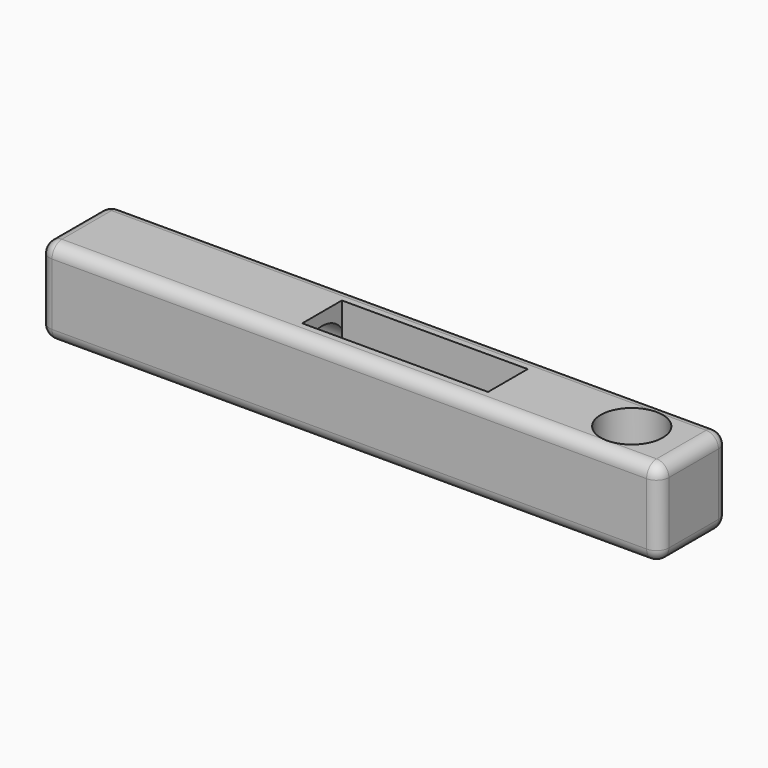
from build123d import *

# Parameters (mm, degrees)
F0_W     = 177.8
F0_H     = 177.8
F1_DEPTH = 1270
F2_R     = 63.5
F3_DEPTH = 177.8
F4_R     = 63.5
F5_DEPTH = 508
F6_R     = 25.4
F7_R     = 25.4
F8_W     = 381
F8_H     = 101.6
F9_DEPTH = 177.8
F10_R    = 25.39999


# Not quite as in the source:
# - a fillet or chamfer is up to 0.001 mm smaller than in the source, because OpenCascade refuses the exact size


with BuildPart() as f1:
    # F0 (on Right) → F1 (new body)
    with BuildSketch(Plane.YZ):
        Rectangle(F0_W, F0_H)
    extrude(amount=F1_DEPTH)

    # F2 (on face) → F3 (cut)
    with BuildSketch(Plane.XY.offset(88.9)):
        with Locations((1143, 0)):
            Circle(F2_R)
    extrude(amount=-F3_DEPTH, mode=Mode.SUBTRACT)

    # F4 (on face) → F5 (cut)
    with BuildSketch(Plane(origin=(0, 0, 0), x_dir=(0, -1, 0), z_dir=(-1, 0, 0))):
        Circle(F4_R)
    extrude(amount=-F5_DEPTH, mode=Mode.SUBTRACT)

    # F6
    f6_edges = [f1.edges().sort_by_distance(p)[0] for p in [
        (635, -88.9, 88.9),
        (635, 88.9, 88.9),
        (635, -88.9, -88.9),
        (635, 88.9, -88.9),
    ]]
    fillet(f6_edges, radius=F6_R)

    # F7
    f7_edges = [f1.edges().sort_by_distance(p)[0] for p in [
        (1270, 0, 88.9),
    ]]
    fillet(f7_edges, radius=F7_R)

    # F8 (on face) → F9 (cut)
    with BuildSketch(Plane.XY.offset(88.9)):
        with Locations((698.5, 0)):
            Rectangle(F8_W, F8_H)
    extrude(amount=-F9_DEPTH, mode=Mode.SUBTRACT)

    # F10 (radius 25.4 in the source; OpenCascade refuses exactly that, so slightly less here)
    f10_edges = [f1.edges().sort_by_distance(p)[0] for p in [
        (0, 0, 88.9),
    ]]
    fillet(f10_edges, radius=F10_R)


solid = f1.part
